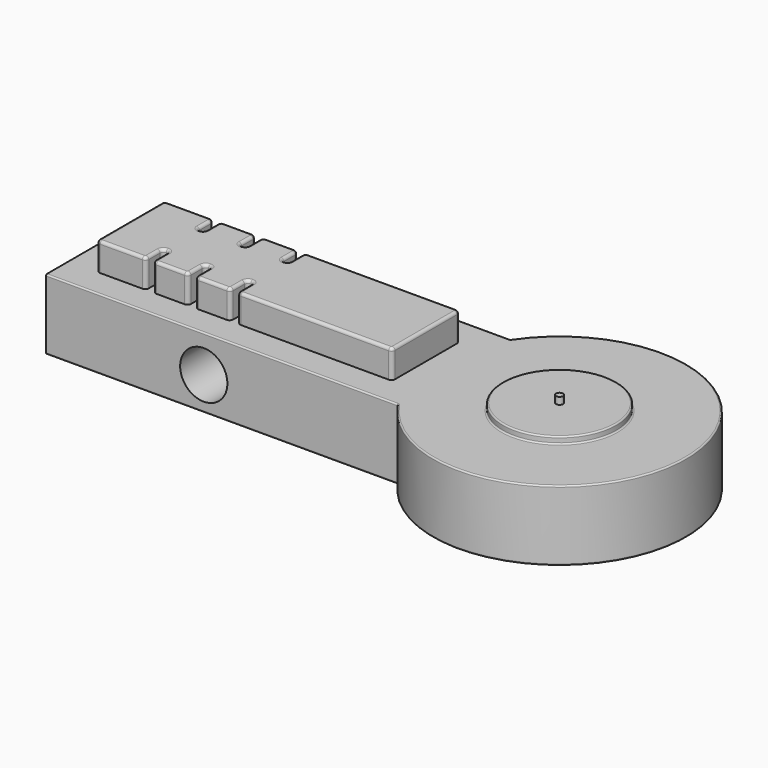
from build123d import *

# Parameters (mm, degrees)
F0_W      = 250
F0_H      = 100
F1_DEPTH  = 50
F3_DEPTH  = 20
F4_R      = 40.3789988007
F5_DEPTH  = 5
F6_R      = 2.5
F7_DEPTH  = 5
F8_R      = 1
F9_R      = 2.49999
F10_R     = 2
F11_R     = 16.7821791649
F12_DEPTH = 140.1397819866


# Not quite as in the source:
# - a fillet or chamfer is up to 0.001 mm smaller than in the source, because OpenCascade refuses the exact size


with BuildPart() as f1:
    # F0 (on Top) → F1 (new body)
    with BuildSketch(Plane.XY):
        with Locations((125, 50)):
            Rectangle(F0_W, F0_H)
        with BuildLine():
            Line((250, 100), (250, 0))
            ThreePointArc((250, 0), (415.1387818866, 50), (250, 100))
        make_face()
    extrude(amount=F1_DEPTH)

    # F2 (on face) → F3 (join)
    with BuildSketch(Plane.XY.offset(50)):
        Polygon((55, 80), (20, 80), (20, 20), (55, 20), (55, 35), (60, 35), (60, 20), (85, 20), (85, 35), (90, 35), (90, 20), (115, 20), (115, 35), (120, 35), (120, 20), (230, 20), (230, 80), (120, 80), (120, 65), (115, 65), (115, 80), (90, 80), (90, 65), (85, 65), (85, 80), (60, 80), (60, 65), (55, 65), align=None)
    extrude(amount=F3_DEPTH)

    # F4 (on face) → F5 (join)
    with BuildSketch(Plane.XY.offset(50)):
        with Locations((325, 50)):
            Circle(F4_R)
    extrude(amount=F5_DEPTH)

    # F6 (on face) → F7 (join)
    with BuildSketch(Plane.XY.offset(55)):
        with Locations((325, 50)):
            Circle(F6_R)
    extrude(amount=F7_DEPTH)

    # F8
    f8_edges = [f1.edges().sort_by_distance(p)[0] for p in [
        (250, 0, 25),
        (250, 100, 25),
        (415.138782, 50, 0),
        (415.138782, 50, 50),
        (284.621001, 50, 55),
        (284.621001, 50, 50),
        (125, 100, 0),
        (125, 100, 50),
        (125, 0, 0),
        (125, 0, 50),
    ]]
    fillet(f8_edges, radius=F8_R)

    # F9 (radius 2.5 in the source; OpenCascade refuses exactly that, so slightly less here)
    f9_edges = [f1.edges().sort_by_distance(p)[0] for p in [
        (55, 35, 60),
        (55, 20, 60),
        (60, 35, 60),
        (60, 20, 60),
        (85, 20, 60),
        (90, 35, 60),
        (90, 20, 60),
        (115, 20, 60),
        (120, 35, 60),
        (120, 20, 60),
        (85, 35, 60),
        (115, 35, 60),
        (55, 65, 60),
        (55, 80, 60),
        (85, 65, 60),
        (85, 80, 60),
        (115, 65, 60),
        (115, 80, 60),
        (60, 65, 60),
        (60, 80, 60),
        (90, 65, 60),
        (90, 80, 60),
        (120, 65, 60),
        (120, 80, 60),
        (20, 80, 60),
        (20, 20, 60),
        (230, 80, 60),
        (230, 20, 60),
    ]]
    fillet(f9_edges, radius=F9_R)

    # F10
    f10_edges = [f1.edges().sort_by_distance(p)[0] for p in [
        (175, 80, 70),
        (230, 50, 70),
        (37.5, 80, 70),
        (54.26777, 79.26777, 70),
        (20.73223, 79.26777, 70),
        (55, 72.5, 70),
        (20, 50, 70),
        (55.73223, 65.73223, 70),
        (20.73223, 20.73223, 70),
        (57.5, 65, 70),
        (37.5, 20, 70),
        (59.26777, 65.73223, 70),
        (54.26777, 20.73223, 70),
        (60, 72.5, 70),
        (55, 27.5, 70),
        (60.73223, 79.26777, 70),
        (55.73223, 34.26777, 70),
        (72.5, 80, 70),
        (57.5, 35, 70),
        (84.26777, 79.26777, 70),
        (59.26777, 34.26777, 70),
        (85, 72.5, 70),
        (60, 27.5, 70),
        (85.73223, 65.73223, 70),
        (60.73223, 20.73223, 70),
        (87.5, 65, 70),
        (72.5, 20, 70),
        (89.26777, 65.73223, 70),
        (84.26777, 20.73223, 70),
        (90, 72.5, 70),
        (85, 27.5, 70),
        (90.73223, 79.26777, 70),
        (85.73223, 34.26777, 70),
        (102.5, 80, 70),
        (87.5, 35, 70),
        (114.26777, 79.26777, 70),
        (89.26777, 34.26777, 70),
        (115, 72.5, 70),
        (90, 27.5, 70),
        (115.73223, 65.73223, 70),
        (90.73223, 20.73223, 70),
        (117.5, 65, 70),
        (102.5, 20, 70),
        (119.26777, 65.73223, 70),
        (114.26777, 20.73223, 70),
        (120, 72.5, 70),
        (115, 27.5, 70),
        (120.73223, 79.26777, 70),
        (115.73223, 34.26777, 70),
        (117.5, 35, 70),
        (229.26777, 79.26777, 70),
        (119.26777, 34.26777, 70),
        (120, 27.5, 70),
        (229.26777, 20.73223, 70),
        (120.73223, 20.73223, 70),
        (175, 20, 70),
    ]]
    fillet(f10_edges, radius=F10_R)

    # F11 (on face) → F12 (cut, through all)
    with BuildSketch(Plane.XZ):
        with Locations((112.087123096, 23.5663745552)):
            Circle(F11_R)
    extrude(amount=-F12_DEPTH, mode=Mode.SUBTRACT)


solid = f1.part
